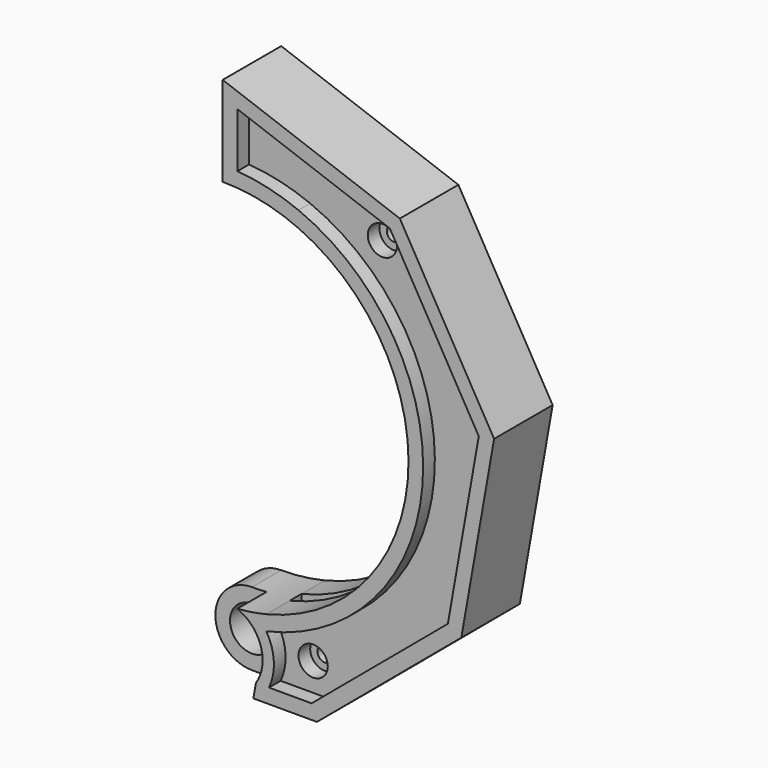
from build123d import *

# Parameters (mm, degrees)
F0_R      = 3
F1_DEPTH  = 5
F2_DEPTH  = 10
F0_R_2    = 2
F3_DEPTH  = 8
F4_DEPTH  = 4
F6_DEPTH  = 4
F0_R_3    = 1
F7_DEPTH  = 6
F9_DEPTH  = 5
F10_DEPTH = 3
F12_DEPTH = 3


with BuildPart() as f1:
    # F0 (on Front) → F1 (new body)
    with BuildSketch(Plane.XZ):
        with BuildLine():
            Line((0, -35.3999999996), (2.6533119314, -35.3999999996))
            ThreePointArc((2.6533119314, -35.3999999996), (4.384153616, -33.1616546164), (5, -30.3999999996))
            ThreePointArc((5, -30.3999999996), (3.5355339059, -26.8644660937), (0, -25.3999999997))
            ThreePointArc((0, -25.3999999997), (-4.9999999999, -30.3999999996), (0, -35.3999999996))
        make_face()
        with Locations((0, -30.3999999996)):
            Circle(F0_R, mode=Mode.SUBTRACT)
    extrude(amount=F1_DEPTH)

    # F0 (on Front) → F2 (join)
    with BuildSketch(Plane.XZ):
        with BuildLine():
            Line((2.6533119314, -35.3999999996), (12.8845462929, -35.3999999996))
            Line((12.8845462929, -35.3999999996), (32.6248164724, -18.8359465726))
            Line((32.6248164724, -18.8359465726), (37.09957244, 6.5416555939))
            Line((37.09957244, 6.5416555939), (24.2150261472, 28.8583444057))
            Line((24.2150261472, 28.8583444057), (0, 37.6718931452))
            Line((0, 37.6718931452), (0, 25.3999999997))
            ThreePointArc((0, 25.3999999997), (5.2987193342, 24.841166909), (10.3642812115, 23.1892577491))
            Line((10.3642812115, 23.1892577491), (10.3642812115, 25.3641809438))
            ThreePointArc((10.3642812115, 25.3641809438), (6.2595477971, 26.6754205469), (2, 27.326909814))
            Line((2, 27.326909814), (2, 34.8155971317))
            Line((2, 34.8155971317), (22.8469455738, 27.2279294674))
            Line((22.8469455738, 27.2279294674), (35.0035513982, 6.1720705321))
            Line((35.0035513982, 6.1720705321), (30.7816065022, -17.7717688002))
            Line((30.7816065022, -17.7717688002), (12.1566058243, -33.3999999997))
            Line((12.1566058243, -33.3999999997), (6.3245553202, -33.3999999997))
            ThreePointArc((6.3245553202, -33.3999999997), (6.9899965839, -30.0259040815), (5.9682330797, -26.7421052628))
            Line((5.9682330797, -26.7421052628), (5.9682330797, -24.6888678131))
            ThreePointArc((5.9682330797, -24.6888678131), (3.0052252445, -25.2215903784), (0, -25.3999999997))
            ThreePointArc((0, -25.3999999997), (3.5355339059, -26.8644660937), (5, -30.3999999996))
            ThreePointArc((5, -30.3999999996), (4.384153616, -33.1616546164), (2.6533119314, -35.3999999996))
        make_face()
    extrude(amount=F2_DEPTH)

    # F0 (on Front) → F3 (join)
    with BuildSketch(Plane.XZ):
        with BuildLine():
            ThreePointArc((10.3642812115, 25.3641809438), (27.3030038884, -2.3034710008), (5.9682330797, -26.7421052628))
            ThreePointArc((5.9682330797, -26.7421052628), (6.9899965839, -30.0259040815), (6.3245553202, -33.3999999997))
            Line((6.3245553202, -33.3999999997), (12.1566058243, -33.3999999997))
            Line((12.1566058243, -33.3999999997), (30.7816065022, -17.7717688002))
            Line((30.7816065022, -17.7717688002), (35.0035513982, 6.1720705321))
            Line((35.0035513982, 6.1720705321), (22.8469455738, 27.2279294674))
            Line((22.8469455738, 27.2279294674), (2, 34.8155971317))
            Line((2, 34.8155971317), (2, 27.326909814))
            ThreePointArc((2, 27.326909814), (6.2595477971, 26.6754205469), (10.3642812115, 25.3641809438))
        make_face()
        with Locations((10.7639788756, -29.5737889045)):
            Circle(F0_R_2, mode=Mode.SUBTRACT)
        with Locations((27.2553512828, -15.7358844)):
            Circle(F0_R_2, mode=Mode.SUBTRACT)
        with Locations((30.9936419152, 5.4650153001)):
            Circle(F0_R_2, mode=Mode.SUBTRACT)
        with Locations((20.2296630396, 24.1087736043)):
            Circle(F0_R_2, mode=Mode.SUBTRACT)
        with Locations((30.9936419152, 5.4650153001)):
            Circle(F0_R_2)
        with Locations((27.2553512828, -15.7358844)):
            Circle(F0_R_2)
    extrude(amount=F3_DEPTH)

    # F0 (on Front) → F4 (join)
    with BuildSketch(Plane.XZ):
        with BuildLine():
            ThreePointArc((10.3642812115, 23.1892577491), (25.2936055675, -2.3223947512), (5.9682330797, -24.6888678131))
            Line((5.9682330797, -24.6888678131), (5.9682330797, -26.7421052628))
            ThreePointArc((5.9682330797, -26.7421052628), (27.3030038884, -2.3034710008), (10.3642812115, 25.3641809438))
            Line((10.3642812115, 25.3641809438), (10.3642812115, 23.1892577491))
        make_face()
    extrude(amount=F4_DEPTH)

    # F5 (on face) → F6 (join)
    with BuildSketch(Plane.XZ.offset(10)):
        with BuildLine():
            ThreePointArc((10.3642812115, 23.1892577491), (25.2936055675, -2.3223947512), (5.9682330797, -24.6888678131))
            Line((5.9682330797, -24.6888678131), (5.9682330797, -26.7421052628))
            ThreePointArc((5.9682330797, -26.7421052628), (27.3030038884, -2.3034710008), (10.3642812115, 25.3641809438))
            Line((10.3642812115, 25.3641809438), (10.3642812115, 23.1892577491))
        make_face()
    extrude(amount=-F6_DEPTH)

    # F0 (on Front) → F7 (join)
    with BuildSketch(Plane.XZ):
        with Locations((20.2296630396, 24.1087736043)):
            Circle(F0_R_2)
        with Locations((20.2296630396, 24.1087736043)):
            Circle(F0_R_3, mode=Mode.SUBTRACT)
        with Locations((10.7639788756, -29.5737889045)):
            Circle(F0_R_2)
        with Locations((10.7639788756, -29.5737889045)):
            Circle(F0_R_3, mode=Mode.SUBTRACT)
    extrude(amount=F7_DEPTH)

    # F8 (on face) → F9 (cut)
    with BuildSketch(Plane.XZ.offset(10)):
        with BuildLine():
            Line((2.6535725711, -35.3997834846), (4.1954981558, -35.3999999996))
            Line((4.1954981558, -35.3999999996), (4.5446208272, -33.4200269408))
            ThreePointArc((4.5446208272, -33.4200269408), (5.2048555211, -28.7618241261), (1.9956840643, -25.3214779407))
            ThreePointArc((1.9956840643, -25.3214779407), (0.9986141145, -25.3803618933), (0, -25.3999999997))
            ThreePointArc((0, -25.3999999997), (3.5355339059, -26.8644660937), (5, -30.3999999996))
            ThreePointArc((5, -30.3999999996), (4.9127701426, -31.4613100854), (4.6534218159, -32.4941346551))
            ThreePointArc((4.6534218159, -32.4941346551), (3.854365705, -34.0852093419), (2.6535725711, -35.3997834846))
        make_face()
        with BuildLine():
            Line((2.6533119314, -35.3999999996), (4.1954981558, -35.3999999996))
            Line((4.1954981558, -35.3999999996), (2.6535725711, -35.3997834846))
            ThreePointArc((2.6535725711, -35.3997834846), (2.6534422527, -35.3998917438), (2.6533119314, -35.3999999996))
        make_face()
        with BuildLine():
            Line((0.0760534773, -35.399421553), (2.6535725711, -35.3997834846))
            ThreePointArc((2.6535725711, -35.3997834846), (3.854365705, -34.0852093419), (4.6534218159, -32.4941346551))
            ThreePointArc((4.6534218159, -32.4941346551), (4.9127701426, -31.4613100854), (5, -30.3999999996))
            ThreePointArc((5, -30.3999999996), (3.5623213911, -33.9085419057), (0.0760534773, -35.399421553))
        make_face()
        with BuildLine():
            ThreePointArc((0, -25.3999999997), (0.9986141145, -25.3803618933), (1.9956840643, -25.3214779407))
            ThreePointArc((1.9956840643, -25.3214779407), (1.0155877723, -25.0387760102), (0, -24.943431372))
            Line((0, -24.943431372), (0, -25.3999999997))
        make_face()
    extrude(amount=-F9_DEPTH, mode=Mode.SUBTRACT)

    # F0 (on Front) → F10 (cut)
    with BuildSketch(Plane.XZ):
        with Locations((20.2296630396, 24.1087736043)):
            Circle(F0_R_2)
        with Locations((20.2296630396, 24.1087736043)):
            Circle(F0_R_3, mode=Mode.SUBTRACT)
        with Locations((10.7639788756, -29.5737889045)):
            Circle(F0_R_2)
        with Locations((10.7639788756, -29.5737889045)):
            Circle(F0_R_3, mode=Mode.SUBTRACT)
    extrude(amount=F10_DEPTH, mode=Mode.SUBTRACT)

    # F11 (on face) → F12 (cut)
    with BuildSketch(Plane.XZ):
        with BuildLine():
            Line((8.3644706756, 32.4991192489), (2, 34.8155971317))
            Line((2, 34.8155971317), (2, 27.326909814))
            ThreePointArc((2, 27.326909814), (5.2188864899, 26.8983870108), (8.3644706756, 26.0920606756))
            Line((8.3644706756, 26.0920606756), (8.3644706756, 32.4991192489))
        make_face()
    extrude(amount=F12_DEPTH, mode=Mode.SUBTRACT)


solid = f1.part
